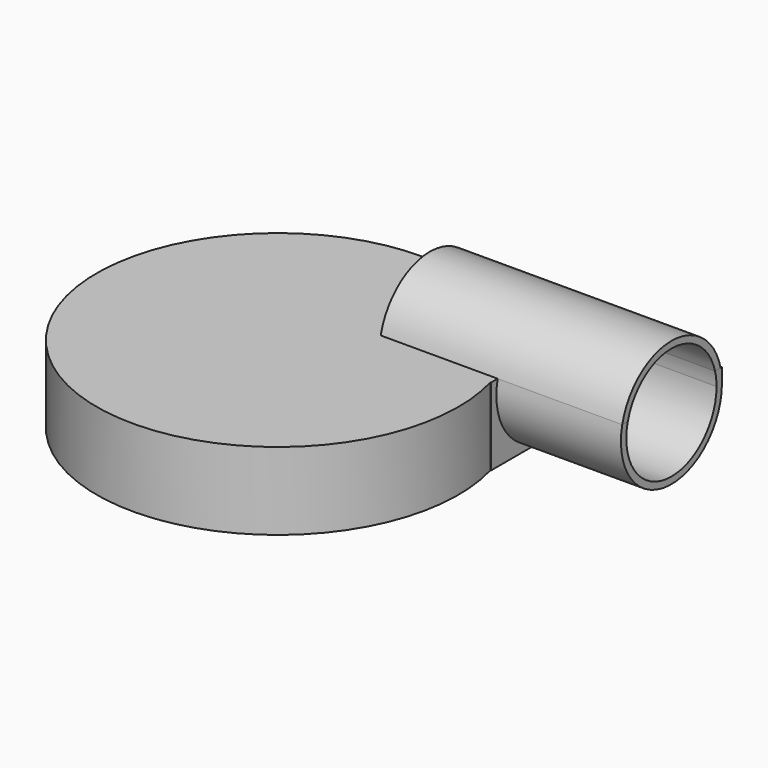
from build123d import *
from build123d import SkipClean  # not in build123d's __all__

# Parameters (mm, degrees)
F1_DEPTH = 46
F3_DEPTH = 74
F4_DEPTH = 143.5


with BuildPart() as f1:
    # F0 (on Top) → F1 (new body)
    with BuildSketch(Plane.XY):
        with BuildLine():
            Line((178, 107.5), (0, 107.5))
            ThreePointArc((0, 107.5), (-65.1632565178, -85.4985379992), (103.6532681588, 28.5))
            Line((103.6532681588, 28.5), (178, 28.5))
            Line((178, 28.5), (178, 107.5))
        make_face()
    extrude(amount=F1_DEPTH)

    # F2 (on face) → F3 (cut)
    with BuildSketch(Plane.YZ.offset(178)):
        with BuildLine():
            ThreePointArc((70, 0), (40.6316496888, 14.1815523673), (33.4760352645, 46))
            Line((33.4760352645, 46), (28.5, 46))
            Line((28.5, 46), (28.5, 0))
            Line((28.5, 0), (70, 0))
        make_face()
        with BuildLine():
            Line((107.5, 0), (107.5, 37.5))
            ThreePointArc((107.5, 37.5), (96.5165042945, 10.9834957055), (70, 0))
            Line((70, 0), (107.5, 0))
        make_face()
        with BuildLine():
            ThreePointArc((37.596296508, 46), (65.714796795, 4.275204538), (103.5, 37.5))
            ThreePointArc((103.5, 37.5), (103.224795462, 41.785203205), (102.403703492, 46))
            Line((102.403703492, 46), (37.596296508, 46))
        make_face()
    extrude(amount=-F3_DEPTH, mode=Mode.SUBTRACT)

    # F2 (on face) → F4 (join)
    with BuildSketch(Plane.YZ.offset(178)):
        with BuildLine():
            ThreePointArc((37.596296508, 46), (70, 71), (102.403703492, 46))
            Line((102.403703492, 46), (106.5239647355, 46))
            ThreePointArc((106.5239647355, 46), (70, 75), (33.4760352645, 46))
            Line((33.4760352645, 46), (37.596296508, 46))
        make_face()
    with SkipClean():  # cleaning this boolean's faces spoils the solid; the shape is the same uncleaned
        extrude(amount=-F4_DEPTH)


solid = f1.part
